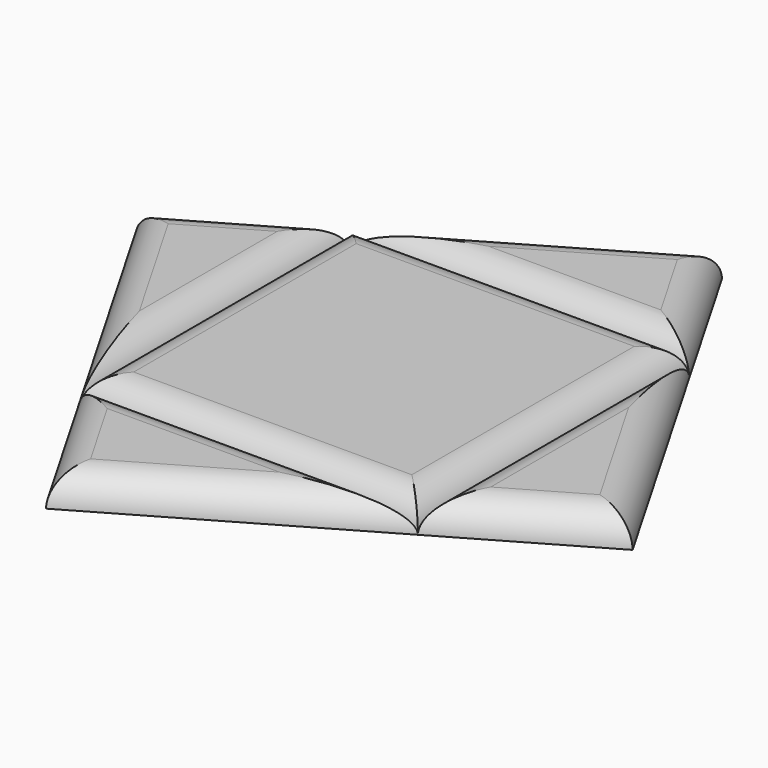
from build123d import *

# Parameters (mm, degrees)
F0_W     = 200
F0_H     = 200
F1_DEPTH = 18
F2_DEPTH = 18
F3_R     = 17.99999
F3_2_R   = 17.99999
F3_3_R   = 17.99999
F3_4_R   = 17.99999
F3_5_R   = 17.99999


# Not quite as in the source:
# - a fillet or chamfer is up to 0.001 mm smaller than in the source, because OpenCascade refuses the exact size


with BuildPart() as f1:
    # F0 (on Top) → F1 (new body)
    with BuildSketch(Plane.XY):
        Rectangle(F0_W, F0_H)
    extrude(amount=F1_DEPTH)

    # F3 (radius 18 in the source; OpenCascade refuses exactly that, so slightly less here)
    f3_edges = [f1.edges().sort_by_distance(p)[0] for p in [
        (0, -100, 18),
        (100, 0, 18),
        (0, 100, 18),
        (-100, 0, 18),
    ]]
    fillet(f3_edges, radius=F3_R)


with BuildPart() as f2:
    # F0 (on Top) → F2 (new body)
    with BuildSketch(Plane.XY):
        Polygon((-186.6025403784, 50), (-100, -100), (-100, 100), align=None)
    extrude(amount=F2_DEPTH)

    # F3#5 (radius 18 in the source; OpenCascade refuses exactly that, so slightly less here)
    f3_5_edges = [f2.edges().sort_by_distance(p)[0] for p in [
        (-100, 0, 18),
        (-143.30127, -25, 18),
        (-143.30127, 75, 18),
    ]]
    fillet(f3_5_edges, radius=F3_5_R)


with BuildPart() as f2b:
    # F0 (on Top) → F2, piece 2 (new body)
    with BuildSketch(Plane.XY):
        Polygon((-100, 100), (100, 100), (50, 186.6025403784), align=None)
    extrude(amount=F2_DEPTH)

    # F3#4 (radius 18 in the source; OpenCascade refuses exactly that, so slightly less here)
    f3_4_edges = [f2b.edges().sort_by_distance(p)[0] for p in [
        (0, 100, 18),
        (-25, 143.30127, 18),
        (75, 143.30127, 18),
    ]]
    fillet(f3_4_edges, radius=F3_4_R)


with BuildPart() as f2c:
    # F0 (on Top) → F2, piece 3 (new body)
    with BuildSketch(Plane.XY):
        Polygon((100, 100), (100, -100), (186.6025403784, -50), align=None)
    extrude(amount=F2_DEPTH)

    # F3#3 (radius 18 in the source; OpenCascade refuses exactly that, so slightly less here)
    f3_3_edges = [f2c.edges().sort_by_distance(p)[0] for p in [
        (100, 0, 18),
        (143.30127, 25, 18),
        (143.30127, -75, 18),
    ]]
    fillet(f3_3_edges, radius=F3_3_R)


with BuildPart() as f2d:
    # F0 (on Top) → F2, piece 4 (new body)
    with BuildSketch(Plane.XY):
        Polygon((-50, -186.6025403784), (100, -100), (-100, -100), align=None)
    extrude(amount=F2_DEPTH)

    # F3#2 (radius 18 in the source; OpenCascade refuses exactly that, so slightly less here)
    f3_2_edges = [f2d.edges().sort_by_distance(p)[0] for p in [
        (0, -100, 18),
        (25, -143.30127, 18),
        (-75, -143.30127, 18),
    ]]
    fillet(f3_2_edges, radius=F3_2_R)


solid = Compound([f1.part, f2.part, f2b.part, f2c.part, f2d.part])
